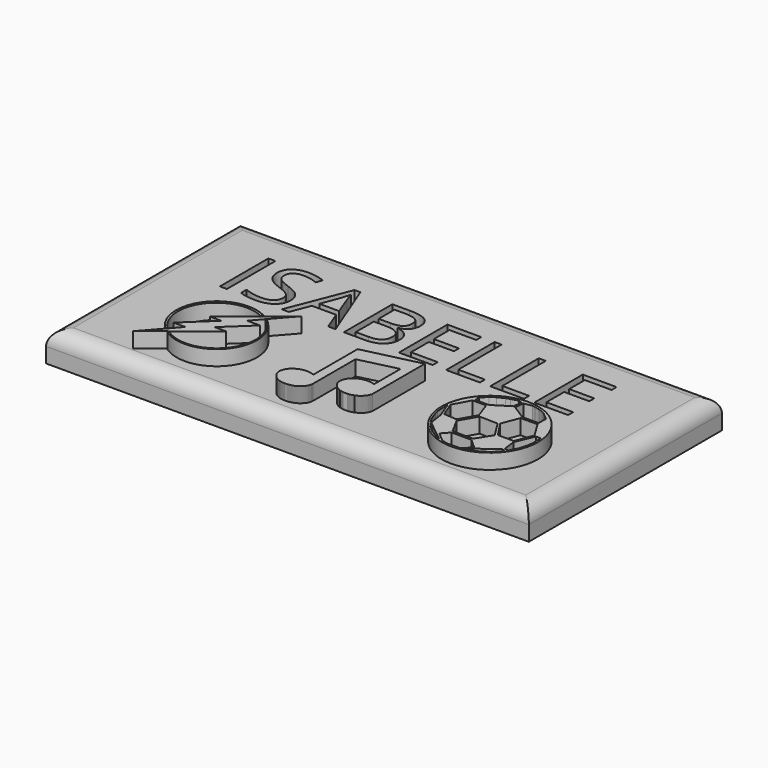
from build123d import *

# Parameters (mm, degrees)
F0_W         = 101.6
F0_H         = 50.8
F1_DEPTH     = 6.35
F2_TEXT_SIZE = 17.8722468575
F3_DEPTH     = 3.175
F5_DEPTH     = 3.175
F6_R         = 10.16
F7_DEPTH     = 3.175
F9_DEPTH     = 3.175
F11_DEPTH    = 3.175
F12_R        = 3.175


# Not quite as in the source:
# - Text() gives the source's letters only with a copy of the font that has no kerning and outlines rounded to 1/6400 em; it was checked with that copy


with BuildPart() as f1:
    # F0 (on Top) → F1 (new body)
    with BuildSketch(Plane.XY):
        with Locations((-0.1096390188, 4.3995542056)):
            Rectangle(F0_W, F0_H)
    extrude(amount=F1_DEPTH)

    # F2 (on face) → F3 (cut)
    with BuildSketch(Plane.XY.offset(6.35)):
        with Locations((-39.8742401847, 8.731531523)):
            Text('ISABELLE', F2_TEXT_SIZE, font='Open Sans', text_align=(TextAlign.LEFT, TextAlign.BOTTOM))
    extrude(amount=-F3_DEPTH, mode=Mode.SUBTRACT)

    # F4 (on face) → F5 (join)
    with BuildSketch(Plane.XY.offset(6.35)):
        Polygon((-29.7351460904, -10.8441486955), (-35.4870669544, -17.3855479807), (-23.5320944339, -7.8745326079), (-25.9289693186, -7.8745326079), (-20.4869601876, -2.7526419202), (-23.1918943486, -2.7526419202), (-17.2162614763, 4.0431749076), (-28.8328845054, -5.4305763915), (-26.4644455165, -5.4305763915), (-32.2163663805, -10.8441486955), align=None)
        with BuildLine():
            ThreePointArc((-31.8574495614, -12.8976395354), (-32.6499405569, -2.5177983958), (-22.5489586592, 0))
            Line((-22.5489586592, 0), (-22.1742205322, 0.3563418868))
            ThreePointArc((-22.1742205322, 0.3563418868), (-33.0158991973, -2.1060781375), (-32.0843048394, -13.184780255))
            Line((-32.0843048394, -13.184780255), (-31.8574495614, -12.8976395354))
        make_face()
        with BuildLine():
            Line((-20.7578404111, -0.548645764), (-20.9479238838, -0.7648190949))
            ThreePointArc((-20.9479238838, -0.7648190949), (-19.4503424584, -11.9934660413), (-30.6112747639, -13.9322420582))
            Line((-30.6112747639, -13.9322420582), (-30.8714255918, -14.1392102063))
            ThreePointArc((-30.8714255918, -14.1392102063), (-19.2471869986, -12.2311734598), (-20.7578404111, -0.548645764))
        make_face()
    extrude(amount=F5_DEPTH)

    # F6 (on face) → F7 (join)
    with BuildSketch(Plane.XY.offset(6.35)):
        with Locations((30.9807900339, -6.6149444319)):
            Circle(F6_R)
    extrude(amount=F7_DEPTH)

    # F8 (on face) → F9 (cut)
    with BuildSketch(Plane.XY.offset(9.525)):
        Polygon((29.9847815186, 0.7865009247), (30.2692968398, 2.5884343777), (29.4437836856, 2.9163651634), (28.0088223517, 2.5032700505), (27.1608904004, 2.2206259891), (25.8563794196, 1.5683706151), (24.8018987477, 0.840018678), (23.687472567, -0.2957078104), (23.687472567, -1.3473678846), (26.5705920756, -1.3473678846), align=None)
        Polygon((30.648496002, 2.5884343777), (30.45187518, 0.6802071002), (33.5405096412, -1.2785748113), (36.9690023363, -1.2785748113), (37.0109155774, 0.6326644798), (36.080442369, 1.3954837341), (35.4685112834, 1.9403545884), (34.9152572453, 2.2085986566), (33.9428707957, 2.5884343777), (32.9704843462, 2.8037654702), (32.3082581162, 2.9163651634), align=None)
        Polygon((37.1037982404, -1.7259202432), (33.5405096412, -1.7633675598), (32.1492440999, -5.3666550666), (34.4253703952, -8.8086182535), (37.7684016114, -8.8086182535), (39.1991473734, -5.145882722), align=None)
        Polygon((34.045348415, -9.1678051417), (31.8183526397, -5.6268707849), (27.9681459069, -5.5290879682), (25.92911385, -9.0618273243), (27.7310479432, -12.3574687168), (32.0224948227, -12.3574687168), align=None)
        Polygon((27.5667160749, -5.2489661612), (26.3293031603, -1.7633675598), (23.4531238675, -1.7633675598), (21.5882919729, -5.1941182464), (22.8315107524, -8.4667112678), (25.5921892822, -8.6678201333), align=None)
        Polygon((22.1990139958, -8.011254837), (21.2592035532, -5.5290879682), (21.3522911072, -8.3088474348), (21.5011592954, -9.0618273243), (21.9333018787, -10.1993799623), (22.1956103342, -10.8898689051), (22.6163975894, -11.6916429251), (22.8094584225, -11.9835899413), (23.0581869051, -11.8891009784), (22.8540729731, -10.7592279091), (22.7078106254, -9.808531031), (22.5981138647, -9.0618273243), align=None)
        Polygon((23.3259554952, -12.3131386936), (23.0581869051, -12.3131386936), (23.3443006873, -12.7381067723), (24.193590501, -13.641811211), (25.0743411823, -14.4260422912), (26.4081824571, -15.2719514444), (27.2872708738, -15.7244242728), (27.593374959, -15.8170068836), (27.6233945042, -15.7696716487), (26.4405012131, -14.8582626134), (25.3804232925, -14.0502760187), (24.5540408885, -13.3635781823), (24.0803919733, -12.9418354481), align=None)
        Polygon((27.8821825235, -12.8461807713), (26.5286434442, -14.3663072959), (28.5775829107, -16.0757359117), (30.0342869014, -16.3475088775), (32.51285851, -16.2931550294), (34.1255226021, -14.6596225232), (32.0888906717, -12.8461807713), align=None)
        Polygon((40.6658612192, -5.2888947539), (39.6316386759, -5.2888947539), (38.0006581545, -9.1370111331), (38.3114628494, -11.8428422138), (39.1707457602, -12.0256682858), (40.0483123958, -10.3070996702), (40.5236668885, -8.606813848), (40.6658612192, -7.6743992977), align=None)
        Polygon((38.8007387519, -12.494280003), (38.1128974259, -12.2600160539), (36.9333587587, -13.1559409201), (35.5517715216, -14.1568882391), (34.353453666, -15.0168566033), (33.3525054157, -16.1023903638), (34.4380401075, -15.7781410962), (35.5940647423, -15.256521292), (36.228466779, -14.9040753022), (36.9333587587, -14.4247487187), (37.5536605716, -13.9313247055), (38.1880663335, -13.3251165971), align=None)
    extrude(amount=-F9_DEPTH, mode=Mode.SUBTRACT)

    # F10 (on face) → F11 (join)
    with BuildSketch(Plane.XY.offset(6.35)):
        Polygon((-2.6907385327, 0.684983097), (-2.6977967937, -10.9809823334), (-2.9570411425, -10.8499024063), (-3.3235852607, -10.7371201739), (-3.6478356924, -10.680728592), (-3.9720861241, -10.6243370101), (-4.296336323, -10.6243370101), (-4.6064890921, -10.6243370101), (-4.9730329774, -10.680728592), (-5.4241642356, -10.7653159648), (-5.8893929236, -10.9344897792), (-6.368719507, -11.1882509664), (-6.8480460905, -11.4984037355), (-7.2286878712, -11.8931438774), (-7.4401558377, -12.1751008555), (-7.6516238041, -12.6262325794), (-7.7362107113, -12.8940911964), (-7.834895514, -13.288830407), (-7.834895514, -13.7258637697), (-7.7362107113, -14.1347013414), (-7.5670364313, -14.529440552), (-7.4303895235, -14.7551419213), (-7.3572566212, -14.8759364308), (-7.2380187921, -15.0296194479), (-7.1034976281, -15.1872010902), (-7.0385516144, -15.2632805649), (-6.8882643245, -15.3985908255), (-6.7191524431, -15.5292684212), (-6.5346667543, -15.6676322222), (-6.3578677364, -15.7983098179), (-6.035017781, -15.9635785967), (-5.7416106574, -16.0880535841), (-5.4156030528, -16.2006746978), (-5.142942071, -16.2510573864), (-4.8791719601, -16.2777304649), (-4.6894894913, -16.2777304649), (-4.5458276847, -16.2922578981), (-4.3856435142, -16.308456113), (-4.2187115178, -16.308456113), (-4.0016048588, -16.308456113), (-3.8667705376, -16.2777304649), (-3.6793735344, -16.2571612746), (-3.494261764, -16.2228830159), (-3.3457153477, -16.1886028945), (-3.18965793, -16.1525894561), (-3.0177446112, -16.1129169445), (-2.8749373741, -16.0651952028), (-2.7634188735, -16.0279291847), (-2.6529482273, -15.991013327), (-2.555973595, -15.9471239895), (-2.4555264972, -15.9030687064), (-2.3674149998, -15.8607754856), (-2.2679272906, -15.8130217217), (-2.2024140477, -15.7733578859), (-2.1401880724, -15.7356842682), (-2.0802014272, -15.6993664134), (-2.0132521167, -15.6534053385), (-1.9572959081, -15.6195276403), (-1.9210556416, -15.58859077), (-1.8910630127, -15.5629872587), (-1.8436253095, -15.5342669392), (-1.787037123, -15.4916150495), (-1.750363037, -15.45389276), (-1.7051553127, -15.4153007285), (-1.6657421058, -15.3816552455), (-1.626719255, -15.3417745605), (-1.5886811263, -15.3093029269), (-1.5520327955, -15.2780177084), (-1.5166973462, -15.2348959818), (-1.4840366133, -15.2015172723), (-1.433061938, -15.1580022247), (-1.4119144762, -15.1290660724), (-1.3794318074, -15.089248307), (-1.3384916803, -15.0474081985), (-1.2971789441, -15.0121411631), (-1.2586833588, -14.9649526702), (-1.222257386, -14.9048315361), (-1.1683354243, -14.8497242151), (-1.1352875736, -14.8010961711), (-1.1080440599, -14.7602306679), (-1.073385668, -14.7082427838), (-1.0490991747, -14.6607995017), (-1.0210798556, -14.6187702836), (-0.9952401328, -14.5682927923), (-0.9621797446, -14.5037098448), (-0.948611431, -14.4644332539), (-0.9217105939, -14.4118828925), (-0.9091912062, -14.3756426578), (-0.8919355532, -14.3256922184), (-0.8561053707, -14.2219735499), (-0.8088523102, -14.0851887448), (-0.7593130268, -13.9417859441), (-0.7463476102, -13.8135709216), (-0.7336127644, -13.6876360137), (-0.7184917817, -13.538104595), (-0.7184917817, -13.4070944041), (-0.7184917817, -13.1808593869), (-0.7184917817, -12.8188813105), (-0.7184917817, -2.3446355481), (7.1561075747, -0.4414265859), (7.2196247056, -0.4383125633), (7.2196247056, -7.3775206693), (7.1293762885, -7.3532294482), (7.0290126289, -7.318558272), (6.9457328399, -7.2897888124), (6.8556360487, -7.2586643822), (6.7581695078, -7.2249940315), (6.6429520957, -7.1987453848), (6.5195956267, -7.1740741841), (6.402702099, -7.1622536248), (6.2659335591, -7.1484232557), (6.163171144, -7.138031669), (6.0448102733, -7.1143595842), (5.8957659639, -7.1143595842), (5.7653607801, -7.1143595842), (5.4833628237, -7.1143595842), (5.296478048, -7.1143595842), (5.229415372, -7.1342778392), (5.1704323851, -7.1463976055), (5.1162973978, -7.1512456052), (5.0387308002, -7.1552856825), (4.9902512692, -7.1593252942), (4.9377321266, -7.1754846722), (4.8876372166, -7.1876044385), (4.8480457626, -7.1940682828), (4.7963345423, -7.1981083602), (4.7567435419, -7.2045721304), (4.7184689471, -7.2108209796), (4.6921046451, -7.2223478928), (4.6628728795, -7.2271203769), (4.6247272179, -7.2333481759), (4.5773703605, -7.2368918918), (4.5056682386, -7.2485982402), (4.4116797978, -7.2896915566), (4.2864183924, -7.3444579354), (4.1635123617, -7.3981945052), (4.0510333442, -7.4165582374), (3.9560773404, -7.4580745885), (3.8625802845, -7.5270598754), (3.766084762, -7.5692493298), (3.6154636981, -7.635103375), (3.4897867444, -7.7278320778), (3.3862931408, -7.8041931554), (3.2948627602, -7.8716535795), (3.1992478236, -7.913458027), (3.1205474323, -7.9715258348), (3.007528824, -8.0549147827), (2.9072628727, -8.1288943894), (2.8706965968, -8.1949615851), (2.7809783351, -8.2946484908), (2.6812916622, -8.4242410958), (2.6164951269, -8.5139591247), (2.536745742, -8.6385682225), (2.4720231123, -8.7396978864), (2.4330992097, -8.800516818), (2.3875667911, -8.8716616126), (2.3480088877, -8.933471176), (2.3274032865, -9.007409215), (2.2758968432, -9.0878884743), (2.2476539016, -9.1768773273), (2.2227321751, -9.2665953562), (2.2055600319, -9.3284149434), (2.1850761758, -9.4021566724), (2.1683918107, -9.462220262), (2.1683918107, -9.5559954643), (2.1472020795, -9.6322783382), (2.1235794723, -9.7173195475), (2.1235794723, -9.8211932927), (2.1024060669, -9.897417394), (2.0769665518, -9.9889994582), (2.0914535854, -10.0777334519), (2.1095777503, -10.1887451043), (2.1235794723, -10.2745065345), (2.1420268682, -10.3874979972), (2.1601117529, -10.4982690561), (2.1751717955, -10.5905127662), (2.205924258, -10.6608496544), (2.2542373654, -10.7713511674), (2.297200961, -10.9089333564), (2.3634283012, -10.9986925152), (2.3874086752, -11.0535403144), (2.4309169196, -11.1530521673), (2.466335019, -11.2340602784), (2.5045055204, -11.2857934763), (2.5681789343, -11.3720912509), (2.6202383451, -11.4212371409), (2.6681036547, -11.4861098945), (2.7128348608, -11.5467349388), (2.7613734179, -11.6125201576), (2.8052084916, -11.653901988), (2.8455825839, -11.692016532), (2.8969435211, -11.7405030387), (2.9472660583, -11.808706119), (3.0031374129, -11.8444635897), (3.054289127, -11.877200507), (3.0946403337, -11.9152934462), (3.1404729481, -11.9585610244), (3.1918334204, -12.0070470922), (3.2377272491, -12.0364189813), (3.2948627602, -12.0729855077), (3.3404483518, -12.1160198878), (3.3876156288, -12.1462067794), (3.4432389843, -12.1818055315), (3.4998439675, -12.218032522), (3.553973278, -12.2521221638), (3.6000947002, -12.275182642), (3.6462161224, -12.3174609616), (3.6878442801, -12.3290243628), (3.7534580731, -12.3472504542), (3.8286502008, -12.3953731518), (3.8825284668, -12.4298550528), (3.9560773404, -12.4769260735), (4.0148258054, -12.4932451255), (4.0579092377, -12.5208183708), (4.1145908118, -12.5365632852), (4.1678999031, -12.5706809163), (4.2086618287, -12.582003697), (4.2613114297, -12.6156992567), (4.3185525574, -12.6156992567), (4.3596301908, -12.6271097341), (4.4044168252, -12.6395504917), (4.481303699, -12.660908001), (4.5497221872, -12.660908001), (4.6564154327, -12.6777794212), (4.6921046451, -12.6876931119), (4.7749634832, -12.722235173), (4.8401653767, -12.7370534465), (4.9025301376, -12.7543770272), (5.0268787891, -12.7666899934), (5.1217172295, -12.7666899934), (5.3202854469, -12.7666899934), (5.5603454821, -12.7666899934), (5.7678050362, -12.7666899934), (5.9752645902, -12.7666899934), (6.0506822849, -12.7543770272), (6.170975219, -12.7347375666), (6.3309092075, -12.7222342417), (6.4087931717, -12.7095186233), (6.520586554, -12.6807419583), (6.6213523969, -12.6570323482), (6.7072999664, -12.6362862065), (6.7839564096, -12.6027707291), (6.9255341661, -12.5796562312), (7.0273806341, -12.5266294926), (7.1103642695, -12.4910650775), (7.19696656, -12.4769260735), (7.2589080155, -12.4312235747), (7.3254154489, -12.4021454139), (7.4050344403, -12.3891465287), (7.496999097, -12.3489380445), (7.5510532324, -12.309055077), (7.6252184707, -12.2766287959), (7.6886589521, -12.2488915577), (7.7760426384, -12.2106859503), (7.8601818532, -12.1561652049), (7.9245509463, -12.1086715131), (7.9885109656, -12.0614796498), (8.0538863317, -12.0132434958), (8.1068351063, -11.9741761009), (8.1675622682, -11.9476251712), (8.1996653444, -11.8974638393), (8.2414467381, -11.853205515), (8.29773581, -11.7935794523), (8.3584786466, -11.7487613351), (8.4166881023, -11.6871010424), (8.4756873436, -11.6246041431), (8.5329422727, -11.5752788261), (8.5976111736, -11.5067761521), (8.6508588707, -11.4503717664), (8.6916456946, -11.3866420043), (8.7431663495, -11.3320670452), (8.7785555565, -11.2767711058), (8.81445634, -11.2206758236), (8.8663965742, -11.1395187622), (8.913438926, -11.0660146841), (8.9414657252, -10.9651184165), (8.9843956411, -10.8980400548), (9.0424717548, -10.807295629), (9.0645109482, -10.7279546977), (9.0907512805, -10.6334896973), (9.1197565198, -10.5528002605), (9.1731026769, -10.4253608733), (9.1857718245, -10.2974151464), (9.1857718245, -10.1645551622), (9.1857718245, 3.508022055), align=None)
    extrude(amount=F11_DEPTH)

    # F12
    f12_edges = [f1.edges().sort_by_distance(p)[0] for p in [
        (-50.909639, 4.399554, 6.35),
        (-0.109639, 29.799554, 6.35),
        (50.690361, 4.399554, 6.35),
        (-0.109639, -21.000446, 6.35),
    ]]
    fillet(f12_edges, radius=F12_R)


solid = f1.part
